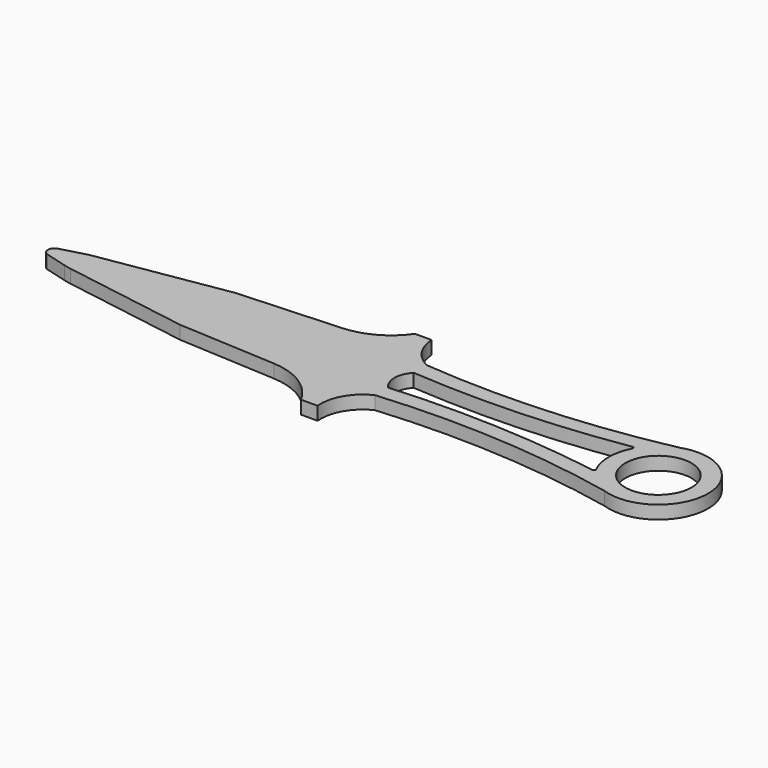
from build123d import *

# Parameters (mm, degrees)
F0_R        = 10
F1_DEPTH    = 4
F2_R        = 0.5
F3_T1_DEPTH = 40.2304088715
F4_T1_DEPTH = 4
F5_SIZE     = 20
F6_R        = 20


# Not quite as in the source:
# - a fillet or chamfer that OpenCascade refuses, or shapes differently, is made with other operations: its cross-section is extruded or revolved along the edge and cut away or added


with BuildPart() as f1:
    # F0 (on Top) → F1 (new body)
    with BuildSketch(Plane.XY):
        with BuildLine():
            Line((50, 20.5837816147), (50, 12.9642039537))
            Line((50, 12.9642039537), (-16.1380209029, 9.3462867662))
            Line((-16.1380209029, 9.3462867662), (-50, 0))
            Line((-50, 0), (-16.1380209029, -9.3462867662))
            Line((-16.1380209029, -9.3462867662), (50, -12.9642039537))
            Line((50, -12.9642039537), (50, -22.5))
            Line((50, -22.5), (55, -22.5))
            ThreePointArc((55, -22.5), (56.5936558821, -15.0125045804), (62.1990375221, -9.7988663689))
            ThreePointArc((62.1990375221, -9.7988663689), (98.7587484272, -9.3015269429), (135, -14.1421356237))
            ThreePointArc((135, -14.1421356237), (155, 0), (135, 14.1421356237))
            ThreePointArc((135, 14.1421356237), (98.7587484272, 9.3015269429), (62.1990375221, 9.7988663689))
            ThreePointArc((62.1990375221, 9.7988663689), (57.1204966078, 14.2040620862), (55, 20.5837816147))
            Line((55, 20.5837816147), (50, 20.5837816147))
        make_face()
        with BuildLine():
            ThreePointArc((62.1990375221, -4.8343795659), (60.2509894701, 0), (62.1990375221, 4.8343795659))
            ThreePointArc((62.1990375221, 4.8343795659), (94.7590329876, 4.3577585856), (127.1470964452, 7.7332315503))
            ThreePointArc((127.1470964452, 7.7332315503), (125, 0), (127.1470964452, -7.7332315503))
            ThreePointArc((127.1470964452, -7.7332315503), (94.7590329876, -4.3577585856), (62.1990375221, -4.8343795659))
        make_face(mode=Mode.SUBTRACT)
        with Locations((140, 0)):
            Circle(F0_R, mode=Mode.SUBTRACT)
    extrude(amount=F1_DEPTH)

    # F2
    f2_edges = [f1.edges().sort_by_distance(p)[0] for p in [
        (127.147096, 7.733232, 2),
        (127.147096, -7.733232, 2),
    ]]
    fillet(f2_edges, radius=F2_R)

    # F3: fillet of radius 2 on 1 edges, made by hand

    # F3_s2 → F3_t1 (cut)
    with BuildSketch(Plane.XY.offset(-18.1152044358)):
        with BuildLine():
            ThreePointArc((-43.0150978282, 1.9279114946), (-44.4829725902, 0), (-43.0150978282, -1.9279114946))
            Line((-43.0150978282, -1.9279114946), (-50, 0))
            Line((-50, 0), (-43.0150978282, 1.9279114946))
        make_face()
    extrude(amount=F3_T1_DEPTH, mode=Mode.SUBTRACT)

    # F4: fillet of radius 20 on 2 edges, made by hand

    # F4_s2 → F4_t1 (join)
    with BuildSketch(Plane.XY):
        with BuildLine():
            ThreePointArc((34.7404872131, 12.1294699712), (43.3406010629, 14.6051902372), (50, 20.5837816147))
            Line((50, 20.5837816147), (50, 12.9642039537))
            Line((50, 12.9642039537), (34.7404872131, 12.1294699712))
        make_face()
        with BuildLine():
            ThreePointArc((50, -22.5), (43.1146209861, -15.1332813357), (33.5101814977, -12.0621691338))
            Line((33.5101814977, -12.0621691338), (50, -12.9642039537))
            Line((50, -12.9642039537), (50, -22.5))
        make_face()
    extrude(amount=F4_T1_DEPTH)

    # F5
    f5_edges = [f1.edges().sort_by_distance(p)[0] for p in [
        (-16.138021, -9.346287, 2),
        (-16.138021, 9.346287, 2),
    ]]
    chamfer(f5_edges, length=F5_SIZE)

    # F6
    f6_edges = [f1.edges().sort_by_distance(p)[0] for p in [
        (-35.417136, 4.025034, 2),
        (-35.417136, -4.025034, 2),
    ]]
    fillet(f6_edges, radius=F6_R)


solid = f1.part
